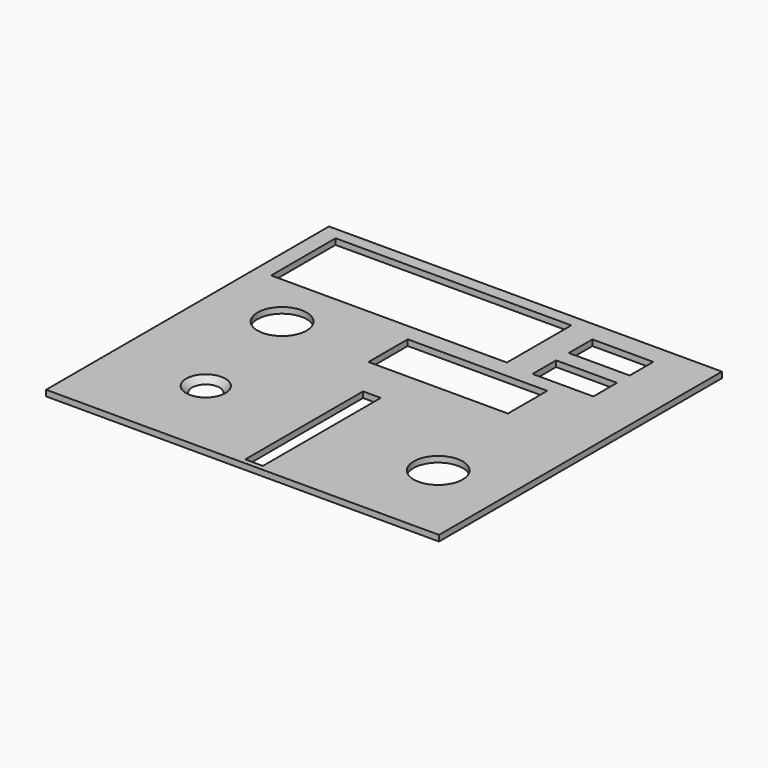
from build123d import *

# Parameters (mm, degrees)
F0_W           = 200
F0_H           = 180
F0_W_2         = 9
F0_H_2         = 75
F0_W_3         = 120
F0_H_3         = 41
F0_W_4         = 71
F0_H_4         = 25
F0_W_5         = 31
F0_H_5         = 15
F1_DEPTH       = 3
F4_D           = 8.8
F4_CSINK_D     = 20
F4_CSINK_ANGLE = 90
F5_D           = 25
F6_D           = 25


# Not quite as in the source:
# - a feature of the source that left no trace in its solid (it failed there, or was rolled back) is left out
# - the program builds the solid bodies; features that only make, move or delete a surface that nothing else refers to are left out


with BuildPart() as f1:
    # F0 (on Top) → F1 (new body)
    with BuildSketch(Plane.XY):
        with Locations((0.7408946753, -7.6781137288)):
            Rectangle(F0_W, F0_H)
        with Locations((4.5, -57.5837731361)):
            Rectangle(F0_W_2, F0_H_2, mode=Mode.SUBTRACT)
        with Locations((-30.8628822118, 55.5105576217)):
            Rectangle(F0_W_3, F0_H_3, mode=Mode.SUBTRACT)
        with Locations((21.3823994361, 13.5011318373)):
            Rectangle(F0_W_4, F0_H_4, mode=Mode.SUBTRACT)
        with Locations((58.7239102691, 41.1898118258)):
            Rectangle(F0_W_5, F0_H_5, mode=Mode.SUBTRACT)
        with Locations((58.7239102691, 64.3030141294)):
            Rectangle(F0_W_5, F0_H_5, mode=Mode.SUBTRACT)
    extrude(amount=F1_DEPTH)

    # F4 (through all)
    with Locations(Plane.XY.offset(3)):
        with Locations((-51.7591053247, -55.4611310363)):
            CounterSinkHole(F4_D / 2, F4_CSINK_D / 2, counter_sink_angle=F4_CSINK_ANGLE)

    # F5 (through all)
    with Locations(Plane.XY.offset(3)):
        with Locations((65.8319948756, -54.5700079396)):
            Hole(F5_D / 2)

    # F6 (through all)
    with Locations(Plane.XY.offset(3)):
        with Locations((-62.68462408, 6.748889561)):
            Hole(F6_D / 2)


solid = f1.part
